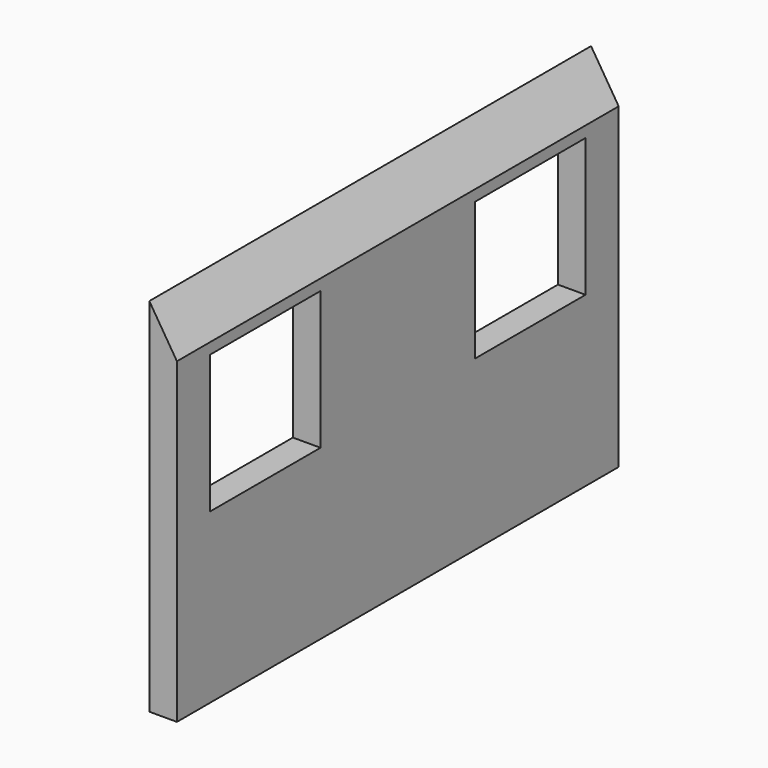
from build123d import *

# Parameters (mm, degrees)
F0_W        = 40
F0_H        = 26.199
F0_W_2      = 10
F0_H_2      = 10
F1_DEPTH    = 2
F2_T1_DEPTH = 56.5405413216


# Not quite as in the source:
# - a fillet or chamfer that OpenCascade refuses, or shapes differently, is made with other operations: its cross-section is extruded or revolved along the edge and cut away or added


with BuildPart() as f1:
    # F0 (on Right) → F1 (new body)
    with BuildSketch(Plane.YZ):
        Rectangle(F0_W, F0_H)
        with Locations((-12, 4.0995)):
            Rectangle(F0_W_2, F0_H_2, mode=Mode.SUBTRACT)
        with Locations((12, 4.0995)):
            Rectangle(F0_W_2, F0_H_2, mode=Mode.SUBTRACT)
    extrude(amount=F1_DEPTH)

    # F2: chamfer of 3.199 x 2.005940846 on 1 edges, made by hand

    # F2_s2 → F2_t1 (cut)
    with BuildSketch(Plane.XZ.offset(-28.2702706608)):
        Polygon((-0.005940846, 13.0995), (2, 9.9005), (2, 13.0995), align=None)
    extrude(amount=F2_T1_DEPTH, mode=Mode.SUBTRACT)


solid = f1.part
